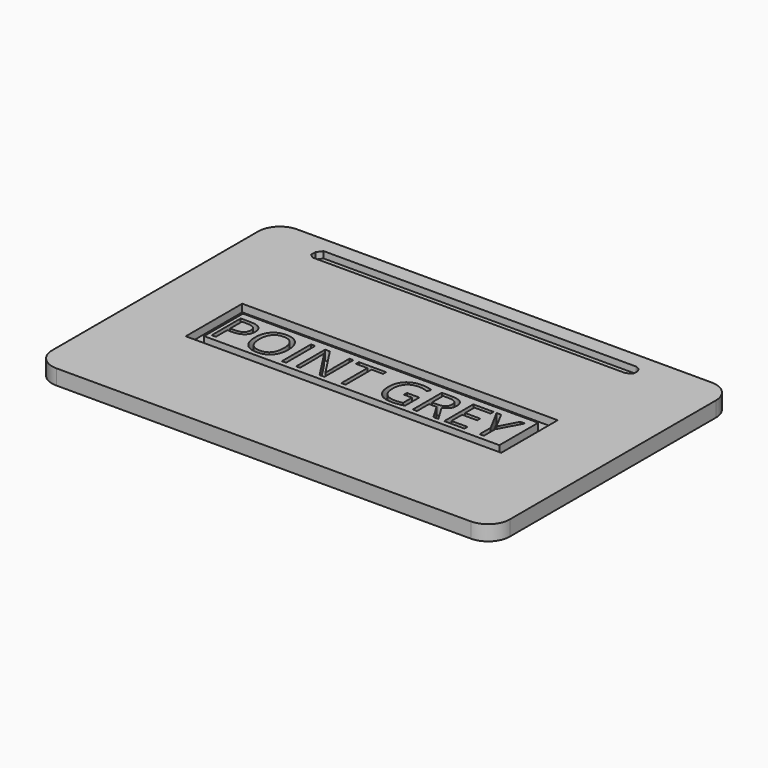
from build123d import *

# Parameters (mm, degrees)
F1_DEPTH     = 3.556
F3_START     = 2.032
F3_DEPTH     = 10.414
F5_START     = 1.778
F4_W         = 73.9320218563
F4_H         = 16.5487378836
F4_W_2       = 69.2038163543
F4_H_2       = 11.3906897604
F5_DEPTH     = 10.414
F7_START     = 1.27
F6_TEXT_SIZE = 11.91950683
F7_DEPTH     = 11.938


# Not quite as in the source:
# - Text() gives the source's letters only with a copy of the font that has no kerning and outlines rounded to 1/6400 em; it was checked with that copy


with BuildPart() as f1:
    # F0 (on Top) → F1 (new body)
    with BuildSketch(Plane.XY):
        with BuildLine():
            Line((51.7577077579, 37.1631160378), (-45.3452463579, 37.1631160378))
            ThreePointArc((-45.3452463579, 37.1631160378), (-48.9373488063, 35.6752184863), (-50.4252463579, 32.0831160378))
            Line((-50.4252463579, 32.0831160378), (-50.4252463579, -28.2939332855))
            ThreePointArc((-50.4252463579, -28.2939332855), (-48.9373488063, -31.8860357339), (-45.3452463579, -33.3739332855))
            Line((-45.3452463579, -33.3739332855), (51.7577077579, -33.3739332855))
            ThreePointArc((51.7577077579, -33.3739332855), (55.3498102064, -31.8860357339), (56.8377077579, -28.2939332855))
            Line((56.8377077579, -28.2939332855), (56.8377077579, 32.0831160378))
            ThreePointArc((56.8377077579, 32.0831160378), (55.3498102064, 35.6752184863), (51.7577077579, 37.1631160378))
        make_face()
    extrude(amount=F1_DEPTH)

    # F2 (on Top) → F3 (cut)
    with BuildSketch(Plane.XY.offset(F3_START)):
        Polygon((37.005610764, 33.4592945874), (-36.1760780215, 33.4592945874), (-37.1209233999, 32.1935229003), (-37.1209233999, 30.9122623876), (-36.1760780215, 30.2033238113), (37.005610764, 30.2033238113), (38.0182228982, 30.5944625288), (38.4582541883, 31.2300622463), (38.4582541883, 32.1590155363), (38.0182228982, 33.0390781164), align=None)
    extrude(amount=F3_DEPTH, mode=Mode.SUBTRACT)

    # F4 (on Top) → F5 (cut)
    with BuildSketch(Plane.XY.offset(F5_START)):
        with Locations((2.1590851247, -0.3945175558)):
            Rectangle(F4_W, F4_H)
        with Locations((2.3740045726, -0.8243550546)):
            Rectangle(F4_W_2, F4_H_2, mode=Mode.SUBTRACT)
    extrude(amount=F5_DEPTH, mode=Mode.SUBTRACT)

    # F6 (on Top) → F7 (cut)
    with BuildSketch(Plane.XY.offset(F7_START)):
        with Locations((-32.5392271756, -5.3738071769)):
            Text('POINT GREY', F6_TEXT_SIZE, font='Open Sans', text_align=(TextAlign.LEFT, TextAlign.BOTTOM))
    extrude(amount=F7_DEPTH, mode=Mode.SUBTRACT)


solid = f1.part
